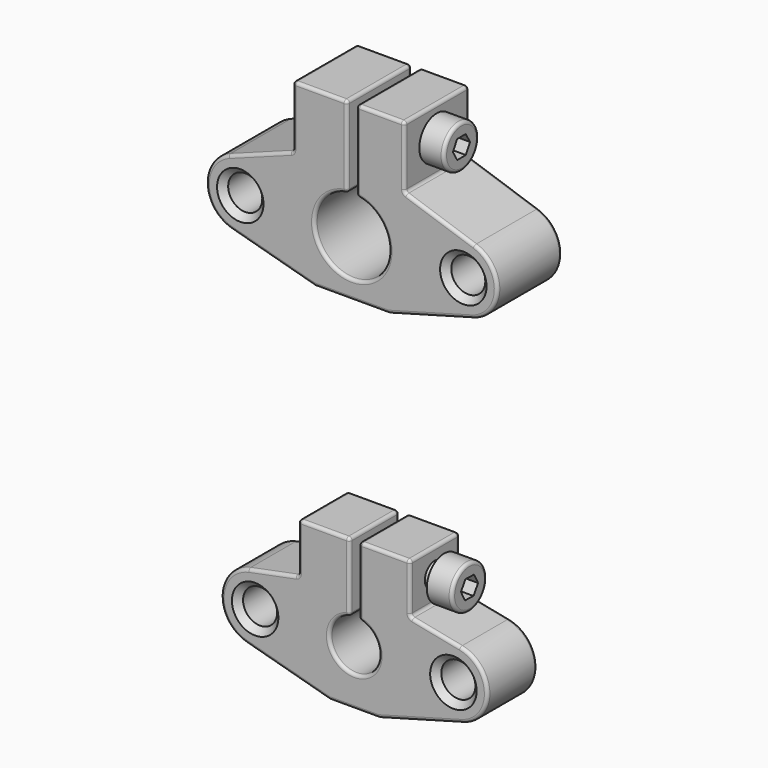
from build123d import *

# Parameters (mm, degrees)
F1_R      = 2.75
F2_DEPTH  = 10
F3_R      = 2
F4_DEPTH  = 21
F3_R_2    = 3.5
F5_DEPTH  = 4.1
F6_SIZE   = 1
F7_R      = 0.5
F8_R      = 2.75
F9_DEPTH  = 13
F10_R     = 2
F11_DEPTH = 21
F10_R_2   = 3.5
F12_DEPTH = 4
F13_SIZE  = 1
F14_R     = 0.5


# Not quite as in the source:
# - a feature names something its author has since deleted; it is built from what else it names


with BuildPart() as f2:
    # F1 (on Front) → F2 (new body)
    with BuildSketch(Plane.XZ):
        with BuildLine():
            ThreePointArc((-8.25, -27.0709415886), (-5.9177929985, -28.4504902432), (-5, -31))
            ThreePointArc((-5, -31), (-11.5495097568, -34.0822070015), (-9.75, -27.0709415886))
            Line((-9.75, -27.0709415886), (-9.75, -16))
            Line((-9.75, -16), (-18.0383976549, -16))
            Line((-18.0383976549, -16), (-18.0383976549, -22.991061002))
            Line((-18.0383976549, -22.991061002), (-18.0383976549, -24))
            Line((-18.0383976549, -24), (-26.07783765, -25.6066461269))
            ThreePointArc((-26.07783765, -25.6066461269), (-30.496551203, -30.8052569044), (-26.4568295288, -36.3035504828))
            Line((-26.4568295288, -36.3035504828), (-13, -40))
            Line((-13, -40), (-5, -40))
            Line((-5, -40), (8.4568295288, -36.3035504828))
            ThreePointArc((8.4568295288, -36.3035504828), (12.4964616393, -30.8027452208), (8.0729081065, -25.6056633221))
            Line((8.0729081065, -25.6056633221), (0, -24))
            Line((0, -24), (0, -20.668335259))
            Line((0, -20.668335259), (0, -16))
            Line((0, -16), (-8.25, -16))
            Line((-8.25, -16), (-8.25, -27.0709415886))
        make_face()
        with Locations((-25, -31)):
            Circle(F1_R, mode=Mode.SUBTRACT)
        with Locations((7, -31)):
            Circle(F1_R, mode=Mode.SUBTRACT)
    extrude(amount=F2_DEPTH)

    # F3 (on offset) → F4 (join)
    with BuildSketch(Plane.YZ.offset(1.5)):
        with Locations((-5, -20)):
            Circle(F3_R)
        Polygon((-4.0765376823, -18.5346613539), (-3.2692483485, -20.0670725035), (-4.1927106662, -21.5324111496), (-5.9234623177, -21.4653386461), (-6.7307516515, -19.9329274965), (-5.8072893338, -18.4675888504), align=None, mode=Mode.SUBTRACT)
        Polygon((-4.1927106662, -21.5324111496), (-3.2692483485, -20.0670725035), (-4.0765376823, -18.5346613539), (-5.8072893338, -18.4675888504), (-6.7307516515, -19.9329274965), (-5.9234623177, -21.4653386461), align=None)
    extrude(amount=-F4_DEPTH)

    # F3 (on offset) → F5 (join)
    with BuildSketch(Plane.YZ.offset(1.5)):
        with Locations((-5, -20)):
            Circle(F3_R_2)
        with Locations((-5, -20)):
            Circle(F3_R, mode=Mode.SUBTRACT)
        with Locations((-5, -20)):
            Circle(F3_R)
        Polygon((-4.0765376823, -18.5346613539), (-3.2692483485, -20.0670725035), (-4.1927106662, -21.5324111496), (-5.9234623177, -21.4653386461), (-6.7307516515, -19.9329274965), (-5.8072893338, -18.4675888504), align=None, mode=Mode.SUBTRACT)
    extrude(amount=F5_DEPTH)

    # F6
    f6_edges = [f2.edges().sort_by_distance(p)[0] for p in [
        (4.25, -10, -31),
        (4.25, 0, -31),
        (-27.75, -10, -31),
        (-27.75, 0, -31),
    ]]
    chamfer(f6_edges, length=F6_SIZE)

    # F7
    f7_edges = [f2.edges().sort_by_distance(p)[0] for p in [
        (-22.058118, -10, -24.803323),
        (-18.038398, -10, -20),
        (-13.894199, -10, -16),
        (-9.75, -10, -21.535471),
        (-8.25, -10, -21.535471),
        (-4.125, -10, -16),
        (0, -10, -20),
        (4.036454, -10, -24.802832),
        (-9, -10, -40),
        (-19.728415, 0, -38.151775),
        (-18.038398, 0, -20),
        (-13.894199, 0, -16),
        (-9.75, 0, -21.535471),
        (-8.25, 0, -21.535471),
        (-4.125, 0, -16),
        (0, 0, -20),
        (4.036454, 0, -24.802832),
        (-9, 0, -40),
        (-18.038398, -5, -24),
        (0, -5, -24),
        (5.6, -8.5, -20),
        (-19.5, -7, -20),
        (-8.25, -5, -16),
        (-9.75, -5, -16),
        (-9, -10, -35),
        (-9, 0, -35),
        (-18.038398, -5, -16),
        (0, -5, -16),
        (-8.25, -5, -27.070942),
        (-9.75, -5, -27.070942),
    ]]
    fillet(f7_edges, radius=F7_R)


with BuildPart() as f9:
    # F8 (on Front) → F9 (new body)
    with BuildSketch(Plane.XZ):
        with BuildLine():
            ThreePointArc((-6.25, 34.9529404499), (-2.5, 32.9686269666), (-1, 29))
            ThreePointArc((-1, 29), (-10.9686269666, 24.5), (-7.75, 34.9529404499))
            Line((-7.75, 34.9529404499), (-7.75, 48))
            Line((-7.75, 48), (-16.5383976549, 48))
            Line((-16.5383976549, 48), (-16.5383976549, 39.008938998))
            Line((-16.5383976549, 39.008938998), (-16.5383976549, 38))
            Line((-16.5383976549, 38), (-26.9106499561, 34.1574622388))
            ThreePointArc((-26.9106499561, 34.1574622388), (-30.4948317819, 28.7616228014), (-26.4568295288, 23.6964495172))
            Line((-26.4568295288, 23.6964495172), (-13, 20))
            Line((-13, 20), (-1, 20))
            Line((-1, 20), (12.4568295288, 23.6964495172))
            ThreePointArc((12.4568295288, 23.6964495172), (16.4978025923, 28.8445437179), (12.7541893916, 34.2127554689))
            Line((12.7541893916, 34.2127554689), (1.5, 38))
            Line((1.5, 38), (1.5, 41.331664741))
            Line((1.5, 41.331664741), (1.5, 48))
            Line((1.5, 48), (-6.25, 48))
            Line((-6.25, 48), (-6.25, 34.9529404499))
        make_face()
        with Locations((-25, 29)):
            Circle(F8_R, mode=Mode.SUBTRACT)
        with Locations((11, 29)):
            Circle(F8_R, mode=Mode.SUBTRACT)
    extrude(amount=F9_DEPTH)

    # F10 (on offset) → F11 (join)
    with BuildSketch(Plane.YZ.offset(1.5)):
        with Locations((-6.5, 43.1584315002)):
            Circle(F10_R)
        Polygon((-5.649158139, 44.6670958524), (-4.7680374147, 43.1759130101), (-5.6188792757, 41.6672486579), (-7.350841861, 41.649767148), (-8.2319625853, 43.1409499903), (-7.3811207243, 44.6496143425), align=None, mode=Mode.SUBTRACT)
        Polygon((-5.6188792757, 41.6672486579), (-4.7680374147, 43.1759130101), (-5.649158139, 44.6670958524), (-7.3811207243, 44.6496143425), (-8.2319625853, 43.1409499903), (-7.350841861, 41.649767148), align=None)
    extrude(amount=-F11_DEPTH)

    # F10 (on offset) → F12 (join)
    with BuildSketch(Plane.YZ.offset(1.5)):
        with Locations((-6.5, 43.1584315002)):
            Circle(F10_R_2)
        with Locations((-6.5, 43.1584315002)):
            Circle(F10_R, mode=Mode.SUBTRACT)
        with Locations((-6.5, 43.1584315002)):
            Circle(F10_R)
        Polygon((-5.649158139, 44.6670958524), (-4.7680374147, 43.1759130101), (-5.6188792757, 41.6672486579), (-7.350841861, 41.649767148), (-8.2319625853, 43.1409499903), (-7.3811207243, 44.6496143425), align=None, mode=Mode.SUBTRACT)
    extrude(amount=F12_DEPTH)

    # F13
    f13_edges = [f9.edges().sort_by_distance(p)[0] for p in [
        (-27.75, -13, 29),
        (8.25, -13, 29),
        (8.25, 0, 29),
        (-27.75, 0, 29),
    ]]
    chamfer(f13_edges, length=F13_SIZE)

    # F14
    f14_edges = [f9.edges().sort_by_distance(p)[0] for p in [
        (-7, 0, 23),
        (-7, 0, 20),
        (5.728415, 0, 21.848225),
        (-19.728415, 0, 21.848225),
        (1.5, 0, 43),
        (5.5, -10, 43.158432),
        (-16.538398, 0, 43),
        (-7.75, 0, 41.47647),
        (-6.25, 0, 41.47647),
        (1.5, -6.5, 48),
        (-6.25, -6.5, 48),
        (-2.375, 0, 48),
        (-2.375, -13, 48),
        (-7.75, -6.5, 48),
        (-16.538398, -6.5, 48),
        (-12.144199, 0, 48),
        (-12.144199, -13, 48),
        (-21.724524, -13, 36.078731),
        (-16.538398, -13, 43),
        (-7, -13, 20),
        (5.728415, -13, 21.848225),
        (1.5, -13, 43),
        (-19.5, -8.5, 43.158432),
        (-6.25, -13, 41.47647),
        (-7.75, -13, 41.47647),
        (-7, -13, 23),
        (-16.538398, -6.5, 38),
        (1.5, -6.5, 38),
        (-6.25, -6.5, 34.95294),
        (-7.75, -6.5, 34.95294),
    ]]
    fillet(f14_edges, radius=F14_R)


solid = Compound([f2.part, f9.part])
